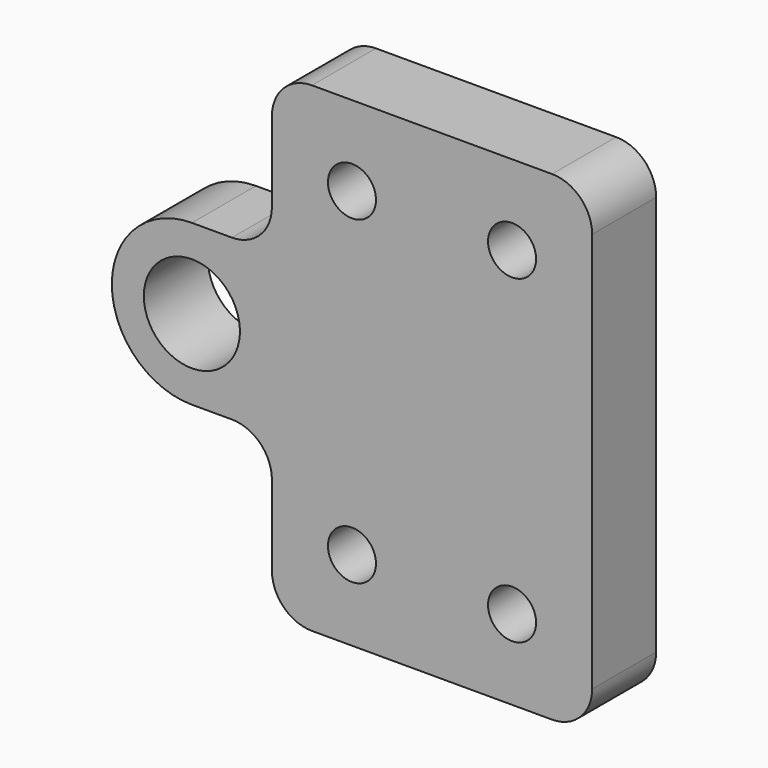
from build123d import *

# Parameters (mm, degrees)
F0_W     = 20
F0_H     = 20
F1_DEPTH = 10
F2_R     = 5
F3_R     = 9.99999
F5_D     = 6
F7_D     = 12


# Not quite as in the source:
# - a fillet or chamfer is up to 0.001 mm smaller than in the source, because OpenCascade refuses the exact size


with BuildPart() as f1:
    # F0 (on Front) → F1 (new body)
    with BuildSketch(Plane.XZ):
        Polygon((-54.7173006759, -1.0133752964), (-14.7173006759, -1.0133752964), (-14.7173006759, 58.9866247036), (-54.7173006759, 58.9866247036), (-54.7173006759, 38.9866247036), (-54.7173006759, 18.9866247036), align=None)
        with Locations((-64.7173006759, 28.9866247036)):
            Rectangle(F0_W, F0_H)
    extrude(amount=F1_DEPTH)

    # F2
    f2_edges = [f1.edges().sort_by_distance(p)[0] for p in [
        (-54.717301, -5, 58.986625),
        (-54.717301, -5, -1.013375),
        (-14.717301, -5, 58.986625),
        (-14.717301, -5, -1.013375),
        (-54.717301, -5, 18.986625),
        (-54.717301, -5, 38.986625),
    ]]
    fillet(f2_edges, radius=F2_R)

    # F3 (radius 10 in the source; OpenCascade refuses exactly that, so slightly less here)
    f3_edges = [f1.edges().sort_by_distance(p)[0] for p in [
        (-74.717301, -5, 38.986625),
        (-74.717301, -5, 18.986625),
    ]]
    fillet(f3_edges, radius=F3_R)

    # F5 (through all)
    with Locations(Plane.XZ.offset(10)):
        with Locations((-44.7173006759, 48.9866247036), (-24.7173006759, 48.9866247036), (-24.7173006759, 8.9866247036), (-44.7173006759, 8.9866247036)):
            Hole(F5_D / 2)

    # F7 (through all)
    with Locations(Plane.XZ.offset(10)):
        with Locations((-64.7173006759, 28.9866247036)):
            Hole(F7_D / 2)


solid = f1.part
